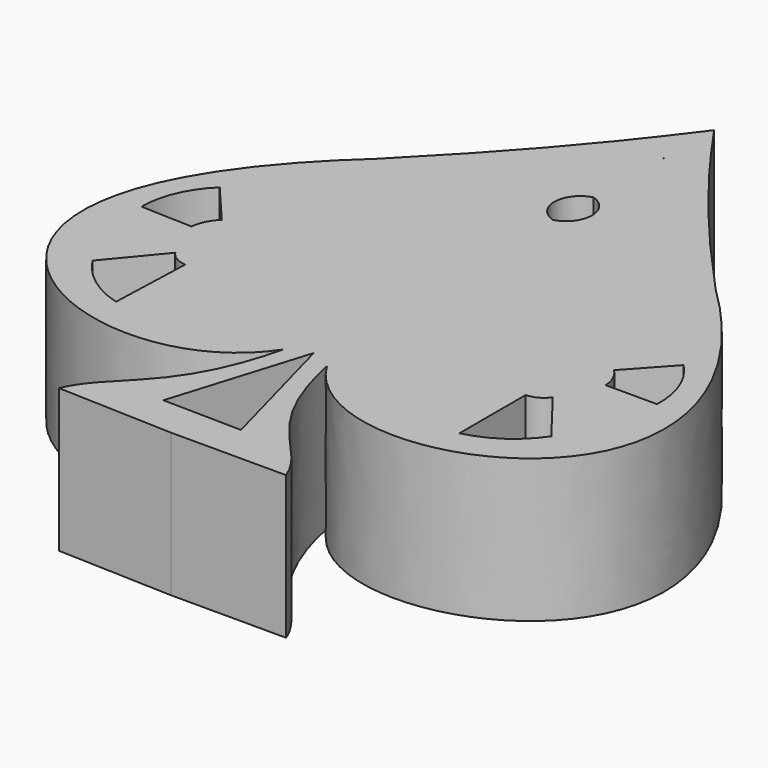
from build123d import *

# Parameters (mm, degrees)
F0_W     = 4.7442697883
F0_H     = 1.9113573674
F0_W_2   = 4.7634891234
F0_H_2   = 1.468620263
F0_W_3   = 4.128358094
F0_H_3   = 1.4289282262
F1_DEPTH = 25.4


# Not quite as in the source:
# - a feature names something its author has since deleted; it is built from what else it names


with BuildPart() as f1:
    # F0 (on Top) → F1 (new body)
    with BuildSketch(Plane.XY):
        with BuildLine():
            Line((-22.9954444695, -37.8900244832), (-2.5283634938, -37.8900244832))
            add(Edge.make_bspline(
                [(-2.5283634938, -37.8900244832), (-5.8608135484, -29.4962804765), (-14.5712196827, -28.3677466214), (-18.5634065419, -8.8018402457)],
                knots=[0, 0, 0, 0, 33.2151331141, 33.2151331141, 33.2151331141, 33.2151331141], degree=3))
            add(Edge.make_bspline(
                [(-18.5634065419, -8.8018402457), (-2.5283634938, -35.3494078415), (62.5428706408, -9.0993279591), (8.9163342491, 43.0122725666)],
                knots=[0, 0, 0, 0, 58.6501358947, 58.6501358947, 58.6501358947, 58.6501358947], degree=3))
            add(Edge.make_bspline(
                [(8.9163342491, 43.0122725666), (-3.4306221642, 56.4400143921), (-11.2726483494, 66.0635232925), (-20.8969525993, 79.9641385674)],
                knots=[0, 0, 0, 0, 47.47917937, 47.47917937, 47.47917937, 47.47917937], degree=3))
            add(Edge.make_bspline(
                [(-52.0068416032, 44.0970606294), (-39.1896790872, 57.0767342864), (-31.0100233031, 66.4149637492), (-20.8969525993, 79.9641385674)],
                knots=[0, 0, 0, 0, 47.47917937, 47.47917937, 47.47917937, 47.47917937], degree=3))
            add(Edge.make_bspline(
                [(-26.3891224094, -8.6624968343), (-43.3591045439, -34.6223823726), (-107.454577438, -6.07238132), (-52.0068416032, 44.0970606294)],
                knots=[0, 0, 0, 0, 58.6501358947, 58.6501358947, 58.6501358947, 58.6501358947], degree=3))
            add(Edge.make_bspline(
                [(-43.4495514732, -37.1613885312), (-39.8203933268, -28.8916017766), (-31.0753324327, -28.0738771005), (-26.3891224094, -8.6624968343)],
                knots=[0, 0, 0, 0, 33.2151331141, 33.2151331141, 33.2151331141, 33.2151331141], degree=3))
            Line((-43.4495514732, -37.1613885312), (-22.9954444695, -37.8900244832))
        make_face()
        Polygon((-29.84915008, -30.9614511052), (-22.4433610347, -6.8842664576), (-15.8994235098, -31.2098376453), (-22.8742867949, -31.0856443752), align=None, mode=Mode.SUBTRACT)
        with BuildLine():
            add(Edge.make_bspline(
                [(-22.3207809169, 0), (-10.655029352, -32.6894562044), (59.6865899861, -11.1531224102), (7.7575119212, 41.9883653522)],
                knots=[0, 0, 0, 0, 51.6500389642, 51.6500389642, 51.6500389642, 51.6500389642], degree=3))
            add(Edge.make_bspline(
                [(-22.3207809169, 0), (-35.1428948343, -32.2534292936), (-104.6732232363, -8.2265585713), (-50.8852053371, 43.0325479438)],
                knots=[0, 0, 0, 0, 51.6500389642, 51.6500389642, 51.6500389642, 51.6500389642], degree=3))
            Line((-50.8852053371, 43.0325479438), (-20.973111277, 75.6869634445))
            Line((-20.973111277, 75.6869634445), (7.7575119212, 41.9883653522))
        make_face(mode=Mode.SUBTRACT)
        with BuildLine():
            add(Edge.make_bspline(
                [(-22.3207809169, 0), (-35.1428948343, -32.2534292936), (-104.6732232363, -8.2265585713), (-50.8852053371, 43.0325479438)],
                knots=[0, 0, 0, 0, 51.6500389642, 51.6500389642, 51.6500389642, 51.6500389642], degree=3))
            add(Edge.make_bspline(
                [(-22.3207809169, 0), (-10.655029352, -32.6894562044), (59.6865899861, -11.1531224102), (7.7575119212, 41.9883653522)],
                knots=[0, 0, 0, 0, 51.6500389642, 51.6500389642, 51.6500389642, 51.6500389642], degree=3))
            Line((7.7575119212, 41.9883653522), (-20.973111277, 75.6869634445))
            Line((-20.973111277, 75.6869634445), (-50.8852053371, 43.0325479438))
        make_face()
        with BuildLine():
            ThreePointArc((-53.4419212435, -11.9822170834), (-59.2752805035, -9.1359017891), (-63.691800004, -4.379438133))
            Line((-63.691800004, -4.379438133), (-56.2167386264, 4.6310161836))
            ThreePointArc((-56.2167386264, 4.6310161836), (-54.7973483092, 3.2789986514), (-52.9181442541, 2.7211345107))
            Line((-52.9181442541, 2.7211345107), (-53.4419212435, -11.9822170834))
        make_face(mode=Mode.SUBTRACT)
        with BuildLine():
            Line((-59.3962358793, 12.1757701265), (-68.5043031466, 12.5002264942))
            ThreePointArc((-68.5043031466, 12.5002264942), (-67.2450849294, 18.6426159936), (-63.6487509213, 23.7788559591))
            Line((-63.6487509213, 23.7788559591), (-57.3389988191, 16.3438184143))
            ThreePointArc((-57.3389988191, 16.3438184143), (-58.7463070002, 14.4467053449), (-59.3962358793, 12.1757701265))
        make_face(mode=Mode.SUBTRACT)
        with BuildLine():
            ThreePointArc((18.8681036234, -5.8494862169), (14.2850517957, -10.4457049841), (8.3540603518, -13.082546182))
            Line((8.3540603518, -13.082546182), (8.3540603518, 1.6301316991))
            ThreePointArc((8.3540603518, 1.6301316991), (10.2519333675, 2.1207418259), (11.7185562849, 3.4213714805))
            Line((11.7185562849, 3.4213714805), (18.8681036234, -5.8494862169))
        make_face(mode=Mode.SUBTRACT)
        with BuildLine():
            ThreePointArc((19.8275279254, 22.2924910486), (23.2387301192, 17.0314760444), (24.2784786969, 10.8481515199))
            Line((24.2784786969, 10.8481515199), (15.1646342129, 10.8481515199))
            ThreePointArc((15.1646342129, 10.8481515199), (14.5959634871, 13.1407849228), (13.2570853457, 15.0867961347))
            Line((13.2570853457, 15.0867961347), (19.8275279254, 22.2924910486))
        make_face(mode=Mode.SUBTRACT)
        with BuildLine():
            add(Edge.make_bspline(
                [(-21.124196495, 69.0203205478), (-22.2645987992, 68.6191021406), (-33.580908588, 63.0681711425), (-30.2861785142, 48.5103170354)],
                knots=[1.924853553, 1.924853553, 1.924853553, 1.924853553, 22.4584134886, 22.4584134886, 22.4584134886, 22.4584134886], degree=3))
            add(Edge.make_bspline(
                [(-21.124196495, 69.0203205478), (-21.1691445632, 69.0500857695), (-21.1554459369, 69.0540761805), (-21.0916213723, 69.0312749979)],
                knots=[0.2728391378, 0.2728391378, 0.2728391378, 0.2728391378, 1.7089042388, 1.7089042388, 1.7089042388, 1.7089042388], degree=3))
            add(Edge.make_bspline(
                [(-21.0594568815, 69.0191678049), (-21.0134776523, 69.04731399), (-21.027025535, 69.0517895479), (-21.0916213723, 69.0312749979)],
                knots=[0.2728391378, 0.2728391378, 0.2728391378, 0.2728391378, 1.7089042388, 1.7089042388, 1.7089042388, 1.7089042388], degree=3))
            add(Edge.make_bspline(
                [(-21.0594568815, 69.0191678049), (-19.9340610017, 68.5776049674), (-8.8225398383, 62.627327695), (-12.633446604, 48.1959953904)],
                knots=[1.924853553, 1.924853553, 1.924853553, 1.924853553, 22.4584134886, 22.4584134886, 22.4584134886, 22.4584134886], degree=3))
            add(Edge.make_bspline(
                [(-12.633446604, 48.1959953904), (-4.4782049954, 44.5908084512), (-1.012446126, 42.8227111697), (4.8599806614, 35.9290093184)],
                knots=[0, 0, 0, 0, 21.3658359252, 21.3658359252, 21.3658359252, 21.3658359252], degree=3))
            Line((4.8599806614, 35.9290093184), (8.7451650402, 35.4348045049))
            Line((8.7451650402, 35.4348045049), (12.5032669737, 31.2499941052))
            add(Edge.make_bspline(
                [(12.5032669737, 31.2499941052), (8.0707731529, 17.1092335792), (6.1978180893, 11.1496476457), (4.9289693125, -2.2719807457)],
                knots=[0, 0, 0, 0, 34.3670304648, 34.3670304648, 34.3670304648, 34.3670304648], degree=3))
            Line((4.9289693125, -2.2719807457), (-17.9089047015, -2.2719807457))
            Line((-17.9089047015, -2.2719807457), (-22.3005021556, 1.1388828675))
            Line((-22.3005021556, 1.1388828675), (-26.8107438558, -2.1134760598))
            Line((-26.8107438558, -2.1134760598), (-49.6341410648, -1.3004389641))
            add(Edge.make_bspline(
                [(-56.0102422262, 32.469934397), (-52.083974651, 18.1803391384), (-50.4243703941, 12.1578530338), (-49.6341410648, -1.3004389641)],
                knots=[0, 0, 0, 0, 34.3670304648, 34.3670304648, 34.3670304648, 34.3670304648], degree=3))
            Line((-56.0102422262, 32.469934397), (-52.105541674, 36.5183021942))
            Line((-52.105541674, 36.5183021942), (-48.2052262113, 36.8738796762))
            add(Edge.make_bspline(
                [(-30.2861785142, 48.5103170354), (-38.5645966004, 45.1977451416), (-42.0911034871, 43.5541509957), (-48.2052262113, 36.8738796762)],
                knots=[0, 0, 0, 0, 21.3658359252, 21.3658359252, 21.3658359252, 21.3658359252], degree=3))
        make_face(mode=Mode.SUBTRACT)
        with BuildLine():
            add(Edge.make_bspline(
                [(-21.0921680822, 69.000571026), (-21.0790768616, 69.0076183464), (-21.0681925114, 69.013820289), (-21.0594568815, 69.0191678049)],
                knots=[0, 0, 0, 0, 0.2728391378, 0.2728391378, 0.2728391378, 0.2728391378], degree=3))
            add(Edge.make_bspline(
                [(-21.0921680822, 69.000571026), (-21.1050001171, 69.0080799317), (-21.1156567762, 69.01466543), (-21.124196495, 69.0203205478)],
                knots=[0, 0, 0, 0, 0.2728391378, 0.2728391378, 0.2728391378, 0.2728391378], degree=3))
            add(Edge.make_bspline(
                [(-21.124196495, 69.0203205478), (-22.2645987992, 68.6191021406), (-33.580908588, 63.0681711425), (-30.2861785142, 48.5103170354)],
                knots=[1.924853553, 1.924853553, 1.924853553, 1.924853553, 22.4584134886, 22.4584134886, 22.4584134886, 22.4584134886], degree=3))
            add(Edge.make_bspline(
                [(-30.2861785142, 48.5103170354), (-38.5645966004, 45.1977451416), (-42.0911034871, 43.5541509957), (-48.2052262113, 36.8738796762)],
                knots=[0, 0, 0, 0, 21.3658359252, 21.3658359252, 21.3658359252, 21.3658359252], degree=3))
            Line((-48.2052262113, 36.8738796762), (-52.105541674, 36.5183021942))
            Line((-52.105541674, 36.5183021942), (-56.0102422262, 32.469934397))
            add(Edge.make_bspline(
                [(-56.0102422262, 32.469934397), (-52.083974651, 18.1803391384), (-50.4243703941, 12.1578530338), (-49.6341410648, -1.3004389641)],
                knots=[0, 0, 0, 0, 34.3670304648, 34.3670304648, 34.3670304648, 34.3670304648], degree=3))
            Line((-49.6341410648, -1.3004389641), (-26.8107438558, -2.1134760598))
            Line((-26.8107438558, -2.1134760598), (-22.3005021556, 1.1388828675))
            Line((-22.3005021556, 1.1388828675), (-17.9089047015, -2.2719807457))
            Line((-17.9089047015, -2.2719807457), (4.9289693125, -2.2719807457))
            add(Edge.make_bspline(
                [(12.5032669737, 31.2499941052), (8.0707731529, 17.1092335792), (6.1978180893, 11.1496476457), (4.9289693125, -2.2719807457)],
                knots=[0, 0, 0, 0, 34.3670304648, 34.3670304648, 34.3670304648, 34.3670304648], degree=3))
            Line((12.5032669737, 31.2499941052), (8.7451650402, 35.4348045049))
            Line((8.7451650402, 35.4348045049), (4.8599806614, 35.9290093184))
            add(Edge.make_bspline(
                [(-12.633446604, 48.1959953904), (-4.4782049954, 44.5908084512), (-1.012446126, 42.8227111697), (4.8599806614, 35.9290093184)],
                knots=[0, 0, 0, 0, 21.3658359252, 21.3658359252, 21.3658359252, 21.3658359252], degree=3))
            add(Edge.make_bspline(
                [(-21.0594568815, 69.0191678049), (-19.9340610017, 68.5776049674), (-8.8225398383, 62.627327695), (-12.633446604, 48.1959953904)],
                knots=[1.924853553, 1.924853553, 1.924853553, 1.924853553, 22.4584134886, 22.4584134886, 22.4584134886, 22.4584134886], degree=3))
        make_face()
        with BuildLine():
            Line((1.5771253966, 0.8908104501), (-22.3005021556, 1.1388828675))
            Line((-22.3005021556, 1.1388828675), (-46.171825282, 1.7410204233))
            add(Edge.make_bspline(
                [(-46.171825282, 1.7410204233), (-45.7708157439, 13.1605637788), (-52.73816584, 22.5929590908), (-52.6217791411, 31.8137129357)],
                knots=[0, 0, 0, 0, 30.7566048147, 30.7566048147, 30.7566048147, 30.7566048147], degree=3))
            Line((-52.6217791411, 31.8137129357), (-47.394574231, 32.6878372218))
            add(Edge.make_bspline(
                [(-47.394574231, 32.6878372218), (-46.4944956501, 34.1402371022), (-39.9368781188, 45.5703020096), (-25.2081565999, 45.257687461)],
                knots=[0, 0, 0, 0, 25.4997698487, 25.4997698487, 25.4997698487, 25.4997698487], degree=3))
            add(Edge.make_bspline(
                [(-25.2081565999, 45.257687461), (-27.3981189013, 47.5347847087), (-28.8692938451, 52.2527268432), (-23.2430618726, 54.7112649227)],
                knots=[0, 0, 0, 0, 9.6556576219, 9.6556576219, 9.6556576219, 9.6556576219], degree=3))
            add(Edge.make_bspline(
                [(-23.2430618726, 54.7112649227), (-23.6007135185, 54.974488922), (-23.6778442933, 55.2155826969), (-23.7461169911, 55.6965485296)],
                knots=[0, 0, 0, 0, 1.1062767458, 1.1062767458, 1.1062767458, 1.1062767458], degree=3))
            Line((-23.7461169911, 55.6965485296), (-26.8019135259, 55.2128791863))
            Line((-26.8019135259, 55.2128791863), (-27.3837317159, 58.8887747819))
            Line((-27.3837317159, 58.8887747819), (-26.355564632, 58.8704674077))
            Line((-26.355564632, 58.8704674077), (-26.287410087, 60.7836866964))
            Line((-26.287410087, 60.7836866964), (-24.6665124446, 60.7548252592))
            Line((-24.6665124446, 60.7548252592), (-24.708365393, 62.4893900249))
            Line((-24.708365393, 62.4893900249), (-23.3507940795, 62.5529359414))
            Line((-23.3507940795, 62.5529359414), (-23.2916032165, 64.2145287318))
            Line((-23.2916032165, 64.2145287318), (-21.1709695666, 64.5749722779))
            Line((-21.1709695666, 64.5749722779), (-19.0645121038, 64.1392618418))
            Line((-19.0645121038, 64.1392618418), (-19.0645121038, 62.4766151085))
            Line((-19.0645121038, 62.4766151085), (-17.7100636065, 62.3647794127))
            Line((-17.7100636065, 62.3647794127), (-17.8136411971, 60.6328041593))
            Line((-17.8136411971, 60.6328041593), (-16.1927435547, 60.6039427221))
            Line((-16.1927435547, 60.6039427221), (-16.1927435547, 58.6895098848))
            Line((-16.1927435547, 58.6895098848), (-15.1645764709, 58.6712025106))
            Line((-15.1645764709, 58.6712025106), (-15.876889146, 55.0183499966))
            Line((-15.876889146, 55.0183499966), (-18.9135298133, 55.6105002761))
            add(Edge.make_bspline(
                [(-19.4513425231, 54.6437501907), (-19.084546715, 54.8940747976), (-18.998881802, 55.1322698593), (-18.9135298133, 55.6105002761)],
                knots=[0, 0, 0, 0, 1.1062767458, 1.1062767458, 1.1062767458, 1.1062767458], degree=3))
            add(Edge.make_bspline(
                [(-17.8240444511, 45.1262071729), (-15.5544048175, 47.323897481), (-13.9162018895, 51.9864745438), (-19.4513425231, 54.6437501907)],
                knots=[0, 0, 0, 0, 9.6556576219, 9.6556576219, 9.6556576219, 9.6556576219], degree=3))
            add(Edge.make_bspline(
                [(3.9008178283, 31.7744798958), (3.0530157965, 33.2580022514), (-3.0935301911, 44.9142754078), (-17.8240444511, 45.1262071729)],
                knots=[0, 0, 0, 0, 25.4997698487, 25.4997698487, 25.4997698487, 25.4997698487], degree=3))
            Line((3.9008178283, 31.7744798958), (9.0935900807, 30.7148192078))
            add(Edge.make_bspline(
                [(1.5771253966, 0.8908104501), (1.5829101903, 12.3173911124), (8.8816406205, 21.4957669377), (9.0935900807, 30.7148192078)],
                knots=[0, 0, 0, 0, 30.7566048147, 30.7566048147, 30.7566048147, 30.7566048147], degree=3))
        make_face(mode=Mode.SUBTRACT)
        with BuildLine():
            Line((-46.171825282, 1.7410204233), (-22.3005021556, 1.1388828675))
            Line((-22.3005021556, 1.1388828675), (1.5771253966, 0.8908104501))
            add(Edge.make_bspline(
                [(1.5771253966, 0.8908104501), (1.5829101903, 12.3173911124), (8.8816406205, 21.4957669377), (9.0935900807, 30.7148192078)],
                knots=[0, 0, 0, 0, 30.7566048147, 30.7566048147, 30.7566048147, 30.7566048147], degree=3))
            Line((9.0935900807, 30.7148192078), (3.9008178283, 31.7744798958))
            add(Edge.make_bspline(
                [(3.9008178283, 31.7744798958), (3.0530157965, 33.2580022514), (-3.0935301911, 44.9142754078), (-17.8240444511, 45.1262071729)],
                knots=[0, 0, 0, 0, 25.4997698487, 25.4997698487, 25.4997698487, 25.4997698487], degree=3))
            add(Edge.make_bspline(
                [(-17.8240444511, 45.1262071729), (-15.5544048175, 47.323897481), (-13.9162018895, 51.9864745438), (-19.4513425231, 54.6437501907)],
                knots=[0, 0, 0, 0, 9.6556576219, 9.6556576219, 9.6556576219, 9.6556576219], degree=3))
            add(Edge.make_bspline(
                [(-19.4513425231, 54.6437501907), (-19.084546715, 54.8940747976), (-18.998881802, 55.1322698593), (-18.9135298133, 55.6105002761)],
                knots=[0, 0, 0, 0, 1.1062767458, 1.1062767458, 1.1062767458, 1.1062767458], degree=3))
            Line((-18.9135298133, 55.6105002761), (-15.876889146, 55.0183499966))
            Line((-15.876889146, 55.0183499966), (-15.1645764709, 58.6712025106))
            Line((-15.1645764709, 58.6712025106), (-16.1927435547, 58.6895098848))
            Line((-16.1927435547, 58.6895098848), (-16.1927435547, 60.6039427221))
            Line((-16.1927435547, 60.6039427221), (-17.8136411971, 60.6328041593))
            Line((-17.8136411971, 60.6328041593), (-17.7100636065, 62.3647794127))
            Line((-17.7100636065, 62.3647794127), (-19.0645121038, 62.4766151085))
            Line((-19.0645121038, 62.4766151085), (-19.0645121038, 64.1392618418))
            Line((-19.0645121038, 64.1392618418), (-21.1709695666, 64.5749722779))
            Line((-21.1709695666, 64.5749722779), (-23.2916032165, 64.2145287318))
            Line((-23.2916032165, 64.2145287318), (-23.3507940795, 62.5529359414))
            Line((-23.3507940795, 62.5529359414), (-24.708365393, 62.4893900249))
            Line((-24.708365393, 62.4893900249), (-24.6665124446, 60.7548252592))
            Line((-24.6665124446, 60.7548252592), (-26.287410087, 60.7836866964))
            Line((-26.287410087, 60.7836866964), (-26.355564632, 58.8704674077))
            Line((-26.355564632, 58.8704674077), (-27.3837317159, 58.8887747819))
            Line((-27.3837317159, 58.8887747819), (-26.8019135259, 55.2128791863))
            Line((-26.8019135259, 55.2128791863), (-23.7461169911, 55.6965485296))
            add(Edge.make_bspline(
                [(-23.2430618726, 54.7112649227), (-23.6007135185, 54.974488922), (-23.6778442933, 55.2155826969), (-23.7461169911, 55.6965485296)],
                knots=[0, 0, 0, 0, 1.1062767458, 1.1062767458, 1.1062767458, 1.1062767458], degree=3))
            add(Edge.make_bspline(
                [(-25.2081565999, 45.257687461), (-27.3981189013, 47.5347847087), (-28.8692938451, 52.2527268432), (-23.2430618726, 54.7112649227)],
                knots=[0, 0, 0, 0, 9.6556576219, 9.6556576219, 9.6556576219, 9.6556576219], degree=3))
            add(Edge.make_bspline(
                [(-47.394574231, 32.6878372218), (-46.4944956501, 34.1402371022), (-39.9368781188, 45.5703020096), (-25.2081565999, 45.257687461)],
                knots=[0, 0, 0, 0, 25.4997698487, 25.4997698487, 25.4997698487, 25.4997698487], degree=3))
            Line((-47.394574231, 32.6878372218), (-52.6217791411, 31.8137129357))
            add(Edge.make_bspline(
                [(-46.171825282, 1.7410204233), (-45.7708157439, 13.1605637788), (-52.73816584, 22.5929590908), (-52.6217791411, 31.8137129357)],
                knots=[0, 0, 0, 0, 30.7566048147, 30.7566048147, 30.7566048147, 30.7566048147], degree=3))
        make_face()
        Polygon((-44.7576590216, 15.5055557954), (-37.679395917, 15.2534070716), (-35.1471528411, 12.5197675079), (-37.679395917, 10.3981904904), (-44.9303970315, 10.6564926543), align=None, mode=Mode.SUBTRACT)
        Polygon((-30.9412721545, 12.0524866506), (-29.4437312744, 13.5210845619), (-27.8865820009, 12.0524866506), (-29.4437312744, 10.525432397), align=None, mode=Mode.SUBTRACT)
        Polygon((-44.3688373522, 8.0533013785), (-22.1914521969, 7.263277148), (0, 7.263277148), (0, 2.287469827), (-22.2800506048, 2.287469827), (-44.5459780059, 3.0806481949), align=None, mode=Mode.SUBTRACT)
        Polygon((-14.8276363188, 10.2651806109), (-16.3294348053, 11.8467019859), (-14.72098995, 13.2589338481), (-13.2766810033, 11.7379538419), align=None, mode=Mode.SUBTRACT)
        Polygon((-9.0568310236, 12.0552075228), (-6.4288745034, 14.6969654201), (0.65387832, 14.6969654201), (0.65387832, 9.8448265344), (-6.6017220804, 9.8448265344), align=None, mode=Mode.SUBTRACT)
        with BuildLine():
            Line((-40.1418328888, 18.7965188536), (-46.5573088461, 19.0250571336))
            ThreePointArc((-46.5573088461, 19.0250571336), (-39.2386461395, 33.6660544705), (-24.1943614945, 40.115172732))
            Line((-24.1943614945, 40.115172732), (-24.3272148478, 32.6539473716))
            Line((-24.3272148478, 32.6539473716), (-26.0486511449, 32.6845989835))
            Line((-26.0486511449, 32.6845989835), (-26.1316949705, 28.0207445723))
            Line((-26.1316949705, 28.0207445723), (-29.55665306, 28.0817288135))
            Line((-29.55665306, 28.0817288135), (-29.6034895982, 25.4513250038))
            Line((-29.6034895982, 25.4513250038), (-29.7527835425, 21.2603784792))
            Line((-29.7527835425, 21.2603784792), (-25.7005311791, 21.1160252323))
            Line((-25.7005311791, 21.1160252323), (-25.7912743076, 18.568704235))
            Line((-25.7912743076, 18.568704235), (-33.0961882413, 17.6953475839))
            Line((-33.0961882413, 17.6953475839), (-35.7368813782, 22.7922350813))
            Line((-35.7368813782, 22.7922350813), (-32.84917873, 25.5710387789))
            Line((-32.84917873, 25.5710387789), (-36.9155790608, 29.7967978759))
            Line((-36.9155790608, 29.7967978759), (-40.934720905, 25.9292229978))
            Line((-40.934720905, 25.9292229978), (-38.0526815829, 22.9342390088))
            Line((-38.0526815829, 22.9342390088), (-40.1418328888, 18.7965188536))
        make_face(mode=Mode.SUBTRACT)
        with BuildLine():
            ThreePointArc((-21.5435338647, 43.6512536062), (-7.2201754113, 40.2072674631), (2.8851975221, 29.4880755246))
            Line((2.8851975221, 29.4880755246), (6.9841672666, 28.7952069193))
            Line((6.9841672666, 28.7952069193), (6.6132862121, 26.9937831908))
            Line((6.6132862121, 26.9937831908), (2.1097264253, 27.6295803487))
            ThreePointArc((2.1097264253, 27.6295803487), (-7.5677131963, 38.4280486782), (-21.5694110126, 42.1979577158))
            ThreePointArc((-21.5694110126, 42.1979577158), (-35.6964434395, 38.9289042288), (-45.7521782087, 28.4818015615))
            Line((-45.7521782087, 28.4818015615), (-50.2755178366, 28.006735892))
            Line((-50.2755178366, 28.006735892), (-50.5820324143, 29.8202212158))
            Line((-50.5820324143, 29.8202212158), (-46.4609945958, 30.3667257165))
            ThreePointArc((-46.4609945958, 30.3667257165), (-35.9804200494, 40.7193676554), (-21.5435338647, 43.6512536062))
        make_face(mode=Mode.SUBTRACT)
        with BuildLine():
            Line((-19.1531257722, 32.5618183913), (-19.0202724189, 40.0230437517))
            ThreePointArc((-19.0202724189, 40.0230437517), (-4.2151153543, 33.0424312338), (2.5776829571, 18.1501675397))
            Line((2.5776829571, 18.1501675397), (-3.8418623153, 18.1501675397))
            Line((-3.8418623153, 18.1501675397), (-5.7823848911, 22.3596394062))
            Line((-5.7823848911, 22.3596394062), (-2.7955498966, 25.250123183))
            Line((-2.7955498966, 25.250123183), (-6.6744568758, 29.2583294213))
            Line((-6.6744568758, 29.2583294213), (-10.888718186, 25.1800144253))
            Line((-10.888718186, 25.1800144253), (-8.101772517, 22.3001688719))
            Line((-8.101772517, 22.3001688719), (-10.9222428873, 17.3005219549))
            Line((-10.9222428873, 17.3005219549), (-18.191434443, 18.4333827347))
            Line((-18.191434443, 18.4333827347), (-18.191434443, 20.9823194891))
            Line((-18.191434443, 20.9823194891), (-14.1366117494, 20.9823194891))
            Line((-14.1366117494, 20.9823194891), (-14.1366117494, 25.1759243172))
            Line((-14.1366117494, 25.1759243172), (-14.0897752112, 27.8063281269))
            Line((-14.0897752112, 27.8063281269), (-17.5147333007, 27.8673123681))
            Line((-17.5147333007, 27.8673123681), (-17.4316894751, 32.5311667793))
            Line((-17.4316894751, 32.5311667793), (-19.1531257722, 32.5618183913))
        make_face(mode=Mode.SUBTRACT)
        with BuildLine():
            ThreePointArc((-21.3630149606, 53.7894412541), (-18.12483498, 49.3327404002), (-21.5196225597, 44.9941450771))
            ThreePointArc((-21.5196225597, 44.9941450771), (-24.7578025403, 49.4508459311), (-21.3630149606, 53.7894412541))
        make_face(mode=Mode.SUBTRACT)
        with BuildLine():
            ThreePointArc((2.5776829571, 18.1501675397), (-4.2151153543, 33.0424312338), (-19.0202724189, 40.0230437517))
            Line((-19.0202724189, 40.0230437517), (-19.1531257722, 32.5618183913))
            Line((-19.1531257722, 32.5618183913), (-17.4316894751, 32.5311667793))
            Line((-17.4316894751, 32.5311667793), (-17.5147333007, 27.8673123681))
            Line((-17.5147333007, 27.8673123681), (-14.0897752112, 27.8063281269))
            Line((-14.0897752112, 27.8063281269), (-14.1366117494, 25.1759243172))
            Line((-14.1366117494, 25.1759243172), (-14.1366117494, 20.9823194891))
            Line((-14.1366117494, 20.9823194891), (-18.191434443, 20.9823194891))
            Line((-18.191434443, 20.9823194891), (-18.191434443, 18.4333827347))
            Line((-18.191434443, 18.4333827347), (-10.9222428873, 17.3005219549))
            Line((-10.9222428873, 17.3005219549), (-8.101772517, 22.3001688719))
            Line((-8.101772517, 22.3001688719), (-10.888718186, 25.1800144253))
            Line((-10.888718186, 25.1800144253), (-6.6744568758, 29.2583294213))
            Line((-6.6744568758, 29.2583294213), (-2.7955498966, 25.250123183))
            Line((-2.7955498966, 25.250123183), (-5.7823848911, 22.3596394062))
            Line((-5.7823848911, 22.3596394062), (-3.8418623153, 18.1501675397))
            Line((-3.8418623153, 18.1501675397), (2.5776829571, 18.1501675397))
        make_face()
        with BuildLine():
            ThreePointArc((-24.1943614945, 40.115172732), (-39.2386461395, 33.6660544705), (-46.5573088461, 19.0250571336))
            Line((-46.5573088461, 19.0250571336), (-40.1418328888, 18.7965188536))
            Line((-40.1418328888, 18.7965188536), (-38.0526815829, 22.9342390088))
            Line((-38.0526815829, 22.9342390088), (-40.934720905, 25.9292229978))
            Line((-40.934720905, 25.9292229978), (-36.9155790608, 29.7967978759))
            Line((-36.9155790608, 29.7967978759), (-32.84917873, 25.5710387789))
            Line((-32.84917873, 25.5710387789), (-35.7368813782, 22.7922350813))
            Line((-35.7368813782, 22.7922350813), (-33.0961882413, 17.6953475839))
            Line((-33.0961882413, 17.6953475839), (-25.7912743076, 18.568704235))
            Line((-25.7912743076, 18.568704235), (-25.7005311791, 21.1160252323))
            Line((-25.7005311791, 21.1160252323), (-29.7527835425, 21.2603784792))
            Line((-29.7527835425, 21.2603784792), (-29.6034895982, 25.4513250038))
            Line((-29.6034895982, 25.4513250038), (-29.55665306, 28.0817288135))
            Line((-29.55665306, 28.0817288135), (-26.1316949705, 28.0207445723))
            Line((-26.1316949705, 28.0207445723), (-26.0486511449, 32.6845989835))
            Line((-26.0486511449, 32.6845989835), (-24.3272148478, 32.6539473716))
            Line((-24.3272148478, 32.6539473716), (-24.1943614945, 40.115172732))
        make_face()
        Polygon((0, 7.263277148), (-22.1914521969, 7.263277148), (-44.3688373522, 8.0533013785), (-44.5459780059, 3.0806481949), (-22.2800506048, 2.287469827), (0, 2.287469827), align=None)
        Polygon((-42.7852563068, 6.1842697226), (-38.6595151567, 6.0372985872), (-38.7103855509, 4.6092761508), (-42.8361267011, 4.7562472863), align=None, mode=Mode.SUBTRACT)
        Polygon((-36.9593330619, 5.8178623416), (-32.1988634885, 5.6482802973), (-32.2511469345, 4.1805909847), (-37.011616508, 4.350173029), align=None, mode=Mode.SUBTRACT)
        Polygon((-30.0360304476, 5.6109514494), (-25.2947680263, 5.4420536208), (-25.3628130835, 3.5319078526), (-30.1040755048, 3.7008056811), align=None, mode=Mode.SUBTRACT)
        with Locations((-16.7828049063, 4.3770501642)):
            Rectangle(F0_W, F0_H, mode=Mode.SUBTRACT)
        with Locations((-9.8661344964, 4.5587262139)):
            Rectangle(F0_W_2, F0_H_2, mode=Mode.SUBTRACT)
        with Locations((-3.7132945145, 4.7373422422)):
            Rectangle(F0_W_3, F0_H_3, mode=Mode.SUBTRACT)
        with BuildLine():
            Line((6.9841672666, 28.7952069193), (2.8851975221, 29.4880755246))
            ThreePointArc((2.8851975221, 29.4880755246), (-7.2201754113, 40.2072674631), (-21.5435338647, 43.6512536062))
            ThreePointArc((-21.5435338647, 43.6512536062), (-35.9804200494, 40.7193676554), (-46.4609945958, 30.3667257165))
            Line((-46.4609945958, 30.3667257165), (-50.5820324143, 29.8202212158))
            Line((-50.5820324143, 29.8202212158), (-50.2755178366, 28.006735892))
            Line((-50.2755178366, 28.006735892), (-45.7521782087, 28.4818015615))
            ThreePointArc((-45.7521782087, 28.4818015615), (-35.6964434395, 38.9289042288), (-21.5694110126, 42.1979577158))
            ThreePointArc((-21.5694110126, 42.1979577158), (-7.5677131963, 38.4280486782), (2.1097264253, 27.6295803487))
            Line((2.1097264253, 27.6295803487), (6.6132862121, 26.9937831908))
            Line((6.6132862121, 26.9937831908), (6.9841672666, 28.7952069193))
        make_face()
        Polygon((0.65387832, 14.6969654201), (-6.4288745034, 14.6969654201), (-3.8528503315, 11.8698262972), (-6.6017220804, 9.8448265344), (0.65387832, 9.8448265344), align=None)
        Polygon((-40.3544344008, 12.5197675079), (-37.679395917, 15.2534070716), (-44.7576590216, 15.5055557954), (-44.9303970315, 10.6564926543), (-37.679395917, 10.3981904904), align=None)
        Polygon((-3.8528503315, 11.8698262972), (-6.4288745034, 14.6969654201), (-9.0568310236, 12.0552075228), (-6.6017220804, 9.8448265344), align=None)
        Polygon((-35.1471528411, 12.5197675079), (-37.679395917, 15.2534070716), (-40.3544344008, 12.5197675079), (-37.679395917, 10.3981904904), align=None)
        with Locations((-16.7828049063, 4.3770501642)):
            Rectangle(F0_W, F0_H)
        Polygon((-25.3628130835, 3.5319078526), (-25.2947680263, 5.4420536208), (-30.0360304476, 5.6109514494), (-30.1040755048, 3.7008056811), align=None)
        with Locations((-9.8661344964, 4.5587262139)):
            Rectangle(F0_W_2, F0_H_2)
        Polygon((-32.2511469345, 4.1805909847), (-32.1988634885, 5.6482802973), (-36.9593330619, 5.8178623416), (-37.011616508, 4.350173029), align=None)
        with Locations((-3.7132945145, 4.7373422422)):
            Rectangle(F0_W_3, F0_H_3)
        Polygon((-38.7103855509, 4.6092761508), (-38.6595151567, 6.0372985872), (-42.7852563068, 6.1842697226), (-42.8361267011, 4.7562472863), align=None)
        Polygon((-14.72098995, 13.2589338481), (-16.3294348053, 11.8467019859), (-14.8276363188, 10.2651806109), (-13.2766810033, 11.7379538419), align=None)
        Polygon((-27.8865820009, 12.0524866506), (-29.4437312744, 13.5210845619), (-30.9412721545, 12.0524866506), (-29.4437312744, 10.525432397), align=None)
    extrude(amount=F1_DEPTH)


solid = f1.part
